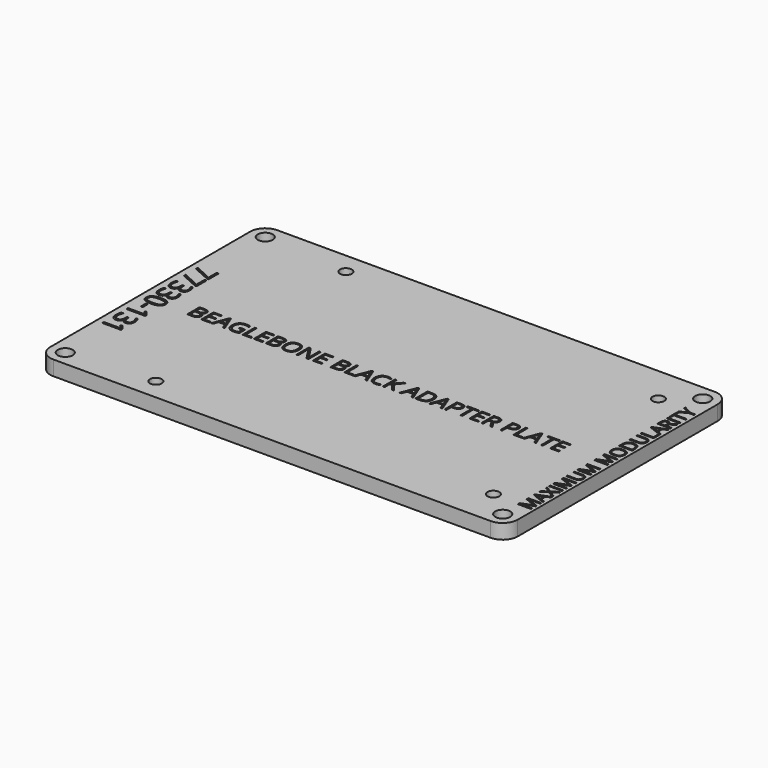
from build123d import *

# Parameters (mm, degrees)
F0_R           = 1.524
F0_R_2         = 1.1938
F1_DEPTH       = 2.9972
F2_TEXT_SIZE   = 5.3613007487
F2_TEXT_SIZE_2 = 4.3810413597
F2_TEXT_SIZE_3 = 3.7383764187
F3_DEPTH       = 0.254


# Not quite as in the source:
# - Text() gives the source's letters only with a copy of the font that has no kerning and outlines rounded to 1/6400 em; it was checked with that copy


with BuildPart() as f1:
    # F0 (on Top) → F1 (new body)
    with BuildSketch(Plane.XY):
        with BuildLine():
            ThreePointArc((0, 3.048), (0.8927385309, 0.8927385309), (3.048, 0))
            Line((3.048, 0), (91.948, 0))
            ThreePointArc((91.948, 0), (94.1032614691, 0.8927385309), (94.996, 3.048))
            Line((94.996, 3.048), (94.996, 53.848))
            ThreePointArc((94.996, 53.848), (94.1032614691, 56.0032614691), (91.948, 56.896))
            Line((91.948, 56.896), (3.048, 56.896))
            ThreePointArc((3.048, 56.896), (0.8927385309, 56.0032614691), (0, 53.848))
            Line((0, 53.848), (0, 3.048))
        make_face()
        with Locations((3.048, 3.048)):
            Circle(F0_R, mode=Mode.SUBTRACT)
        with Locations((20.447, 4.318)):
            Circle(F0_R_2, mode=Mode.SUBTRACT)
        with Locations((91.948, 3.048)):
            Circle(F0_R, mode=Mode.SUBTRACT)
        with Locations((86.487, 7.493)):
            Circle(F0_R_2, mode=Mode.SUBTRACT)
        with Locations((3.048, 53.848)):
            Circle(F0_R, mode=Mode.SUBTRACT)
        with Locations((20.447, 52.578)):
            Circle(F0_R_2, mode=Mode.SUBTRACT)
        with Locations((86.487, 49.403)):
            Circle(F0_R_2, mode=Mode.SUBTRACT)
        with Locations((91.948, 53.848)):
            Circle(F0_R, mode=Mode.SUBTRACT)
    extrude(amount=F1_DEPTH)

    # F2 (on face) → F3 (cut)
    with BuildSketch(Plane.XY.offset(2.9972)):
        with Locations(Location((1.27, 39.7002), (0, 0, -90))):
            Text('77330-131', F2_TEXT_SIZE, font='Open Sans', text_align=(TextAlign.LEFT, TextAlign.BOTTOM))
        with Locations((9.525, 25.4)):
            Text('BEAGLEBONE BLACK ADAPTER PLATE', F2_TEXT_SIZE_2, font='Open Sans', text_align=(TextAlign.LEFT, TextAlign.BOTTOM))
        with Locations(Location((94.361, 6.858), (0, 0, 90))):
            Text('MAXIMUM MODULARITY', F2_TEXT_SIZE_3, font='Open Sans', text_align=(TextAlign.LEFT, TextAlign.BOTTOM))
    extrude(amount=-F3_DEPTH, mode=Mode.SUBTRACT)


solid = f1.part
